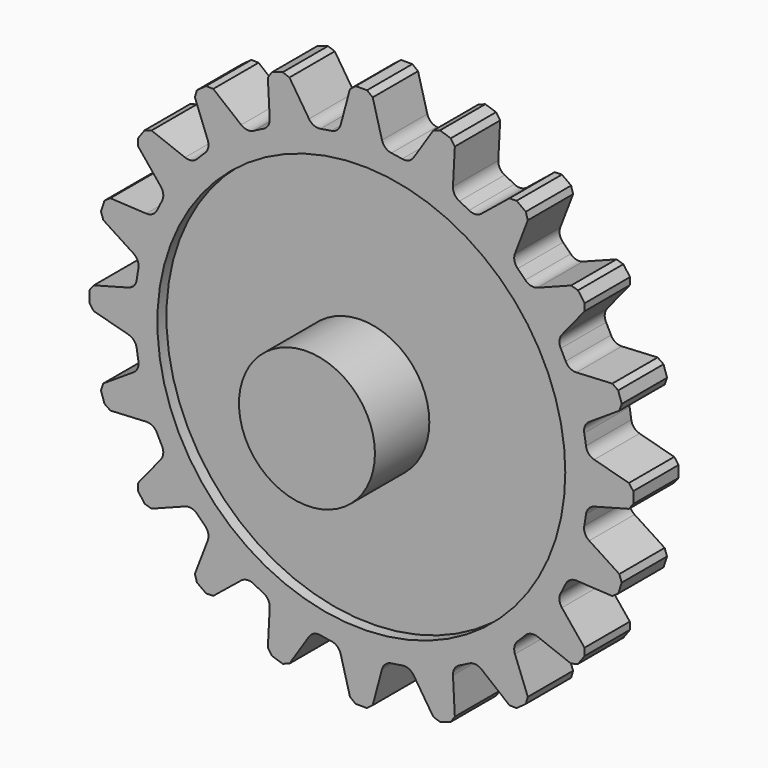
from build123d import *

# Parameters (mm, degrees)
F0_R            = 100
F1_DEPTH        = 25
F3_DEPTH        = 25
F3_COPIES_COUNT = 20
F4_SIZE         = 2
F5_R            = 5
F6_R            = 90
F7_DEPTH        = 5
F8_R            = 30
F9_DEPTH        = 30


# Not quite as in the source:
# - a pattern or mirror of a feature is missing from the dataset's text; its kind, count and spacing are read off the source's solid


with BuildPart() as f1:
    # F0 (on Front) → F1 (new body)
    with BuildSketch(Plane.XZ):
        Circle(F0_R)
    extrude(amount=F1_DEPTH)

    # F2 (on face) → F3 (join)
    with BuildSketch(Plane.XZ.offset(25)):
        with BuildLine():
            Line((9.9931095726, 99.4994359837), (-9.9931095726, 99.4994359837))
            ThreePointArc((-9.9931095726, 99.4994359837), (-67.0846071865, -74.159662072), (100, 0))
            ThreePointArc((100, 0), (74.159662072, 67.0846071865), (9.9931095726, 99.4994359837))
        make_face()
        with BuildLine():
            Line((-4.5, 120), (-9.9931095726, 99.4994359837))
            ThreePointArc((-9.9931095726, 99.4994359837), (0, 100), (9.9931095726, 99.4994359837))
            Line((9.9931095726, 99.4994359837), (4.5, 120))
            Line((4.5, 120), (-4.5, 120))
        make_face()
    f3 = extrude(amount=-F3_DEPTH)

    # F3_copies: F3 ×20 about axis
    f3_copies_axis = Axis((0, 0, 0), (0, 1, 0))
    for i in range(1, F3_COPIES_COUNT):
        add(f3.rotate(f3_copies_axis, i * 360 / F3_COPIES_COUNT))

    # F4
    f4_edges = [f1.edges().sort_by_distance(p)[0] for p in [
        (-4.5, -12.5, 120),
        (4.5, -12.5, 120),
        (-41.361794, -12.5, 112.736205),
        (-66.893654, -12.5, 99.727073),
        (-32.802285, -12.5, 115.517358),
        (-74.174807, -12.5, 94.437006),
        (32.802285, -12.5, 115.517358),
        (41.361794, -12.5, 112.736205),
        (66.893654, -12.5, 99.727073),
        (74.174807, -12.5, 94.437006),
        (94.437006, -12.5, 74.174807),
        (99.727073, -12.5, 66.893654),
        (112.736205, -12.5, 41.361794),
        (115.517358, -12.5, 32.802285),
        (120, -12.5, 4.5),
        (120, -12.5, -4.5),
        (115.517358, -12.5, -32.802285),
        (112.736205, -12.5, -41.361794),
        (99.727073, -12.5, -66.893654),
        (94.437006, -12.5, -74.174807),
        (74.174807, -12.5, -94.437006),
        (66.893654, -12.5, -99.727073),
        (41.361794, -12.5, -112.736205),
        (32.802285, -12.5, -115.517358),
        (4.5, -12.5, -120),
        (-4.5, -12.5, -120),
        (-32.802285, -12.5, -115.517358),
        (-41.361794, -12.5, -112.736205),
        (-66.893654, -12.5, -99.727073),
        (-74.174807, -12.5, -94.437006),
        (-94.437006, -12.5, -74.174807),
        (-99.727073, -12.5, -66.893654),
        (-112.736205, -12.5, -41.361794),
        (-115.517358, -12.5, -32.802285),
        (-120, -12.5, -4.5),
        (-120, -12.5, 4.5),
        (-115.517358, -12.5, 32.802285),
        (-112.736205, -12.5, 41.361794),
        (-99.727073, -12.5, 66.893654),
        (-94.437006, -12.5, 74.174807),
    ]]
    chamfer(f4_edges, length=F4_SIZE)

    # F5
    f5_edges = [f1.edges().sort_by_distance(p)[0] for p in [
        (9.99311, -12.5, 99.499436),
        (-9.99311, -12.5, 99.499436),
        (21.243005, -12.5, 97.717628),
        (-21.243005, -12.5, 97.717628),
        (40.251029, -12.5, 91.541546),
        (50.399706, -12.5, 86.370537),
        (-40.251029, -12.5, 91.541546),
        (-50.399706, -12.5, 86.370537),
        (66.568897, -12.5, 74.622932),
        (74.622932, -12.5, 66.568897),
        (-66.568897, -12.5, 74.622932),
        (-74.622932, -12.5, 66.568897),
        (86.370537, -12.5, 50.399706),
        (91.541546, -12.5, 40.251029),
        (-86.370537, -12.5, 50.399706),
        (-91.541546, -12.5, 40.251029),
        (97.717628, -12.5, 21.243005),
        (99.499436, -12.5, 9.99311),
        (-97.717628, -12.5, 21.243005),
        (-99.499436, -12.5, 9.99311),
        (99.499436, -12.5, -9.99311),
        (97.717628, -12.5, -21.243005),
        (-99.499436, -12.5, -9.99311),
        (-97.717628, -12.5, -21.243005),
        (91.541546, -12.5, -40.251029),
        (86.370537, -12.5, -50.399706),
        (-91.541546, -12.5, -40.251029),
        (-86.370537, -12.5, -50.399706),
        (74.622932, -12.5, -66.568897),
        (66.568897, -12.5, -74.622932),
        (-74.622932, -12.5, -66.568897),
        (-66.568897, -12.5, -74.622932),
        (50.399706, -12.5, -86.370537),
        (40.251029, -12.5, -91.541546),
        (-50.399706, -12.5, -86.370537),
        (-40.251029, -12.5, -91.541546),
        (21.243005, -12.5, -97.717628),
        (9.99311, -12.5, -99.499436),
        (-21.243005, -12.5, -97.717628),
        (-9.99311, -12.5, -99.499436),
    ]]
    fillet(f5_edges, radius=F5_R)

    # F6 (on face) → F7 (cut)
    with BuildSketch(Plane.XZ.offset(25)):
        Circle(F6_R)
    extrude(amount=-F7_DEPTH, mode=Mode.SUBTRACT)


with BuildPart() as f9:
    # F8 (on face) → F9 (new body)
    with BuildSketch(Plane.XZ.offset(25)):
        Circle(F8_R)
    extrude(amount=F9_DEPTH)


solid = Compound([f1.part, f9.part])
